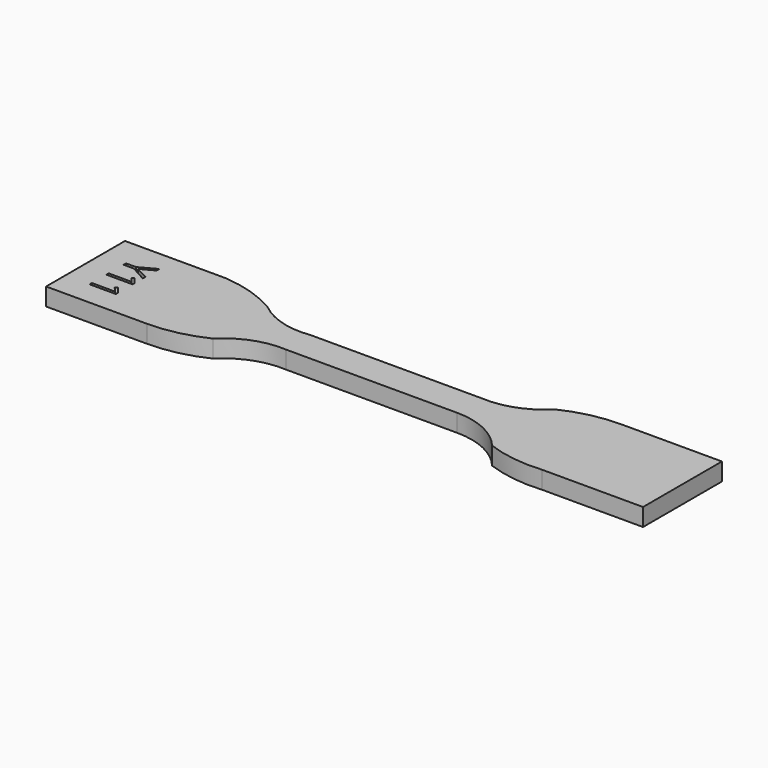
from build123d import *

# Parameters (mm, degrees)
F1_DEPTH     = 3.4
F2_TEXT_SIZE = 7.0564552314
F3_DEPTH     = 1


# Not quite as in the source:
# - Text() gives the source's letters only with a copy of the font that has no kerning and outlines rounded to 1/6400 em; it was checked with that copy


with BuildPart() as f1:
    # F0 (on Top) → F1 (new body)
    with BuildSketch(Plane.XY):
        with BuildLine():
            Line((-14.4320548165, 19.7811394548), (-33.8720548165, 19.7811394548))
            Line((-33.8720548165, 19.7811394548), (-33.8720548165, 0.7811394548))
            Line((-33.8720548165, 0.7811394548), (-14.4320548165, 0.7811394548))
            ThreePointArc((-14.4320548165, 0.7811394548), (-8.9053122052, 1.3996892086), (-3.6520548165, 3.2247301661))
            ThreePointArc((-3.6520548165, 3.2247301661), (1.3014698263, 6.4128780055), (7.1279451835, 7.2811394548))
            Line((7.1279451835, 7.2811394548), (40.1279451835, 7.2811394548))
            ThreePointArc((40.1279451835, 7.2811394548), (46.0837574042, 5.9511158081), (50.9079451835, 2.2137538538))
            ThreePointArc((50.9079451835, 2.2137538538), (56.2191047011, 0.9041953221), (61.6879451835, 0.7811394548))
            Line((61.6879451835, 0.7811394548), (81.1279451835, 0.7811394548))
            Line((81.1279451835, 0.7811394548), (81.1279451835, 19.7811394548))
            Line((81.1279451835, 19.7811394548), (61.6879451835, 19.7811394548))
            ThreePointArc((61.6879451835, 19.7811394548), (56.1612025723, 19.162589701), (50.9079451835, 17.3375487435))
            ThreePointArc((50.9079451835, 17.3375487435), (45.9544205407, 14.1494009041), (40.1279451835, 13.2811394548))
            Line((40.1279451835, 13.2811394548), (7.1279451835, 13.2811394548))
            ThreePointArc((7.1279451835, 13.2811394548), (1.4167452884, 13.6925537245), (-3.6520548165, 16.3560723447))
            ThreePointArc((-3.6520548165, 16.3560723447), (-8.8458057958, 18.686276846), (-14.4320548165, 19.7811394548))
        make_face()
    extrude(amount=F1_DEPTH)

    # F2 (on face) → F3 (cut)
    with BuildSketch(Plane.XY.offset(3.4)):
        with Locations(Location((-29.1824135929, 15.8650862949), (0, 0, -90))):
            Text('Y11', F2_TEXT_SIZE, font='Open Sans', text_align=(TextAlign.LEFT, TextAlign.BOTTOM))
    extrude(amount=-F3_DEPTH, mode=Mode.SUBTRACT)


solid = f1.part
